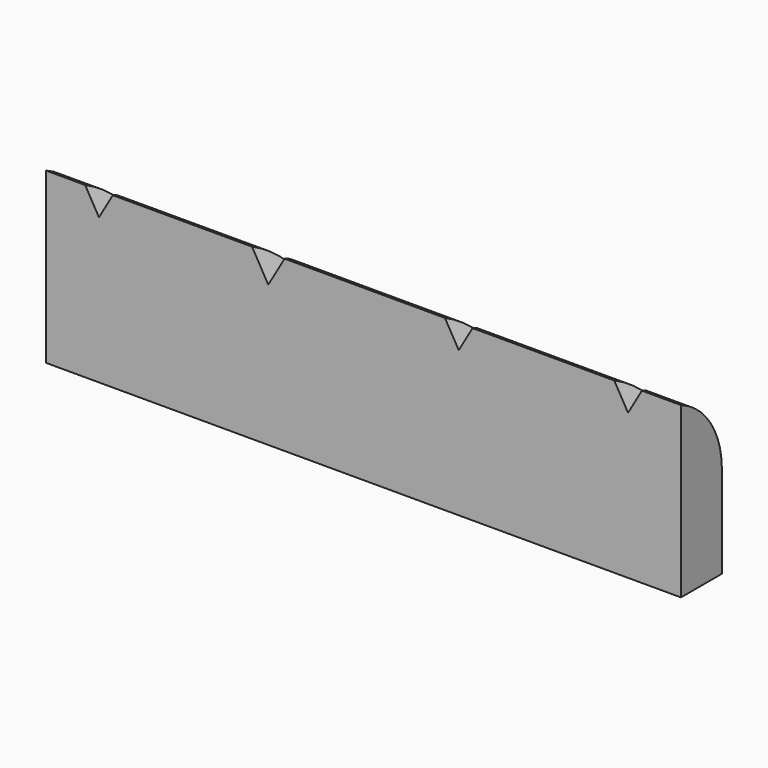
from build123d import *

# Parameters (mm, degrees)
F0_W        = 38.1
F0_H        = 3.0734
F1_DEPTH    = 10.16
F3_T1_DEPTH = 61.4345004446
F4_DEPTH    = 25.4


# Not quite as in the source:
# - a fillet or chamfer that OpenCascade refuses, or shapes differently, is made with other operations: its cross-section is extruded or revolved along the edge and cut away or added


with BuildPart() as f1:
    # F0 (on Top) → F1 (new body)
    with BuildSketch(Plane.XY):
        with Locations((0, 1.5367)):
            Rectangle(F0_W, F0_H)
    extrude(amount=F1_DEPTH)

    # F3: fillet of radius 5.08 on 1 edges, made by hand

    # F3_s2 → F3_t1 (cut)
    with BuildSketch(Plane.YZ.offset(-30.7172502223)):
        with BuildLine():
            ThreePointArc((3.0734, 5.4930999111), (2.2360364445, 8.2870999111), (0, 10.16))
            Line((0, 10.16), (3.0734, 10.16))
            Line((3.0734, 10.16), (3.0734, 5.4930999111))
        make_face()
    extrude(amount=F3_T1_DEPTH, mode=Mode.SUBTRACT)

    # F2 (on face) → F4 (cut)
    with BuildSketch(Plane.XZ):
        Polygon((-15.875, 8.7222954744), (-15.0449409051, 10.16), (-16.7050590949, 10.16), align=None)
        Polygon((-4.7382939367, 10.16), (-6.6917060633, 10.16), (-5.715, 8.4682954744), align=None)
        Polygon((6.5450590949, 10.16), (4.8849409051, 10.16), (5.715, 8.7222954744), align=None)
        Polygon((16.7050590949, 10.16), (15.0449409051, 10.16), (15.875, 8.7222954744), align=None)
    extrude(amount=-F4_DEPTH, mode=Mode.SUBTRACT)


solid = f1.part
